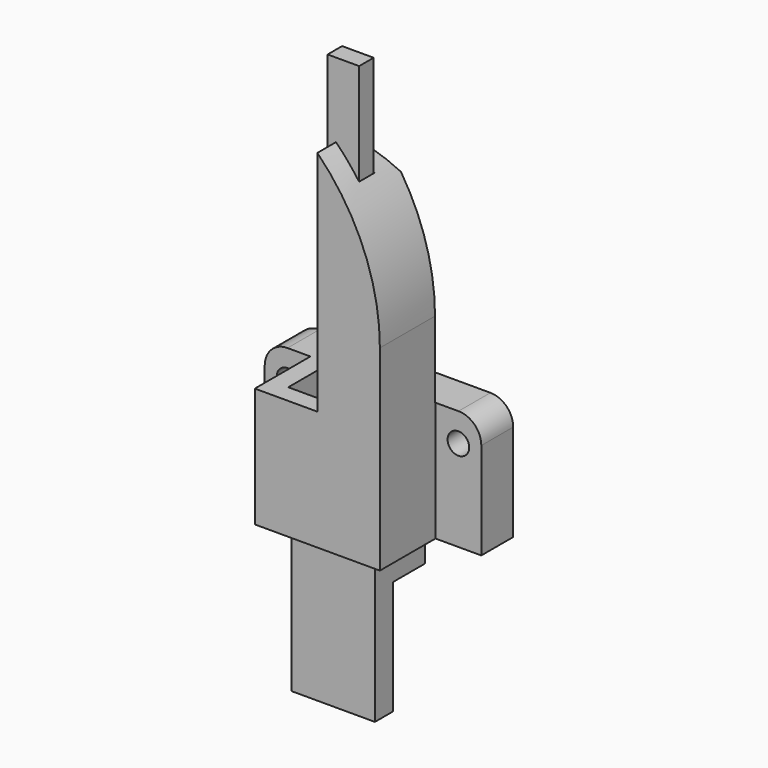
from build123d import *

# Parameters (mm, degrees)
F0_W         = 18.542
F0_H         = 8.89
F1_DEPTH     = 6.35
F2_DEPTH     = 5.08
F3_W         = 18.542
F3_H         = 5.0685656011
F4_DEPTH     = 25.4
F5_W         = 7.493
F5_H         = 4.191
F6_DEPTH     = 125.222
F7_DEPTH     = 6.35
F8_W         = 7.0358
F8_H         = 4.0401988663
F9_DEPTH     = 127
F11_DEPTH    = 21.59
F12_R        = 2.413
F13_DEPTH    = 25.4
F14_W        = 19.3073768169
F14_H        = 14.7933904082
F15_DEPTH    = 41.656
F16_W        = 10.1808982092
F16_H        = 21.59
F16_W_2      = 10.2163404226
F17_DEPTH    = 15.494
F18_DEPTH    = 5.08
F19_DEPTH    = 6.35
F20_W        = 13.9391366392
F20_H        = 15.3644406528
F21_DEPTH    = 50.8
F22_T1_DEPTH = 184.1193966406
F23_SIZE     = 6.35
F24_R        = 5.08
F25_W        = 7.1110432036
F25_H        = 4.2591807432
F26_DEPTH    = 73.152
F27_DEPTH    = 4.445
F28_R        = 2.54
F30_DEPTH    = 25.4
F29_R        = 3.937
F31_DEPTH    = 11.43


# Not quite as in the source:
# - a fillet or chamfer that OpenCascade refuses, or shapes differently, is made with other operations: its cross-section is extruded or revolved along the edge and cut away or added


with BuildPart() as f1:
    # F0 (on Top) → F1 (new body)
    with BuildSketch(Plane.XY):
        Rectangle(F0_W, F0_H)
    extrude(amount=F1_DEPTH)

    # F2 (add): a face of the model
    f2_faces = [f1.faces().sort_by_distance(p)[0] for p in [
        (0, -4.445, 3.175),
    ]]
    extrude(f2_faces, amount=F2_DEPTH)

    # F3 (on face) → F4 (join)
    with BuildSketch(Plane(origin=(0, 0, 0), x_dir=(1, 0, 0), z_dir=(0, 0, -1))):
        with Locations((0, 6.9907171994)):
            Rectangle(F3_W, F3_H)
    extrude(amount=F4_DEPTH)

    # F5 (on face) → F6 (cut)
    with BuildSketch(Plane(origin=(0, 0, -25.4), x_dir=(1, 0, 0), z_dir=(0, 0, -1))):
        with Locations((1.6165795822, 6.5519343989)):
            Rectangle(F5_W, F5_H)
    extrude(amount=-F6_DEPTH, mode=Mode.SUBTRACT)

    # F7 (add): a face of the model
    f7_faces = [f1.faces().sort_by_distance(p)[0] for p in [
        (-0.2230199424, -1.9865219107, 6.35),
    ]]
    extrude(f7_faces, amount=F7_DEPTH)

    # F19 (add): a face of the model
    f19_faces = [f1.faces().sort_by_distance(p)[0] for p in [
        (-0.2230199424, -1.9865219107, 12.7),
    ]]
    extrude(f19_faces, amount=F19_DEPTH)

    # F28 (on face) → F30 (cut)
    with BuildSketch(Plane.XY.offset(19.05)):
        Circle(F28_R)
    extrude(amount=-F30_DEPTH, mode=Mode.SUBTRACT)

    # F29 (on face) → F31 (cut)
    with BuildSketch(Plane.XY.offset(19.05)):
        Circle(F29_R)
    extrude(amount=-F31_DEPTH, mode=Mode.SUBTRACT)


with BuildPart() as f9:
    # F8 (on face) → F9 (new body)
    with BuildSketch(Plane(origin=(0, 0, -25.4), x_dir=(1, 0, 0), z_dir=(0, 0, -1))):
        with Locations((1.5412379404, 6.6265871283)):
            Rectangle(F8_W, F8_H)
    extrude(amount=-F9_DEPTH)


with BuildPart() as f11:
    # F10 (on face) → F11 (new body)
    with BuildSketch(Plane.XY.offset(12.7)):
        Polygon((-24.13, 5.969), (-24.13, 0), (-24.13, -13.97), (24.1554770619, -13.97), (24.1554770619, 5.969), align=None)
    extrude(amount=F11_DEPTH)

    # F12 (on face) → F13 (cut)
    with BuildSketch(Plane(origin=(0, 5.969, 0), x_dir=(-1, 0, 0), z_dir=(0, 1, 0))):
        with Locations((19.05, 27.94)):
            Circle(F12_R)
        with Locations((-19.05, 27.94)):
            Circle(F12_R)
    extrude(amount=-F13_DEPTH, mode=Mode.SUBTRACT)

    # F14 (on face) → F15 (cut)
    with BuildSketch(Plane(origin=(0, 0, 12.7), x_dir=(1, 0, 0), z_dir=(0, 0, -1))):
        with Locations((-0.0584181398, 2.5467472151)):
            Rectangle(F14_W, F14_H)
    extrude(amount=-F15_DEPTH, mode=Mode.SUBTRACT)

    # F16 (on face) → F17 (cut)
    with BuildSketch(Plane.XZ.offset(13.97)):
        with Locations((-19.0395508954, 23.495)):
            Rectangle(F16_W, F16_H)
        with Locations((19.0473068506, 23.495)):
            Rectangle(F16_W_2, F16_H)
    extrude(amount=-F17_DEPTH, mode=Mode.SUBTRACT)

    # F18 (add): a face of the model
    f18_faces = [f11.faces().sort_by_distance(p)[0] for p in [
        (19.0473068506, 2.0464031983, 12.7),
    ]]
    extrude(f18_faces, amount=F18_DEPTH)

    # F20 (on face) → F21 (join)
    with BuildSketch(Plane.XY.offset(34.29)):
        with Locations((6.9695683196, -6.2877796736)):
            Rectangle(F20_W, F20_H)
    extrude(amount=F21_DEPTH)

    # F22: fillet of radius 47.8303990977 on 1 edges, made by hand

    # F22_s2 → F22_t1 (cut)
    with BuildSketch(Plane.XZ.offset(-85.7719186467)):
        with BuildLine():
            ThreePointArc((0, 85.09), (10.3172191212, 69.5970819282), (13.9391366392, 51.3390088024))
            Line((13.9391366392, 51.3390088024), (13.9391366392, 85.09))
            Line((13.9391366392, 85.09), (0, 85.09))
        make_face()
    extrude(amount=F22_T1_DEPTH, mode=Mode.SUBTRACT)

    # F23
    f23_edges = [f11.edges().sort_by_distance(p)[0] for p in [
        (0, 1.394441, 59.69),
    ]]
    chamfer(f23_edges, length=F23_SIZE)

    # F24
    f24_edges = [f11.edges().sort_by_distance(p)[0] for p in [
        (-24.13, 3.7465, 34.29),
        (24.155477, 3.7465, 34.29),
    ]]
    fillet(f24_edges, radius=F24_R)

    # F25 (on face) → F26 (cut)
    with BuildSketch(Plane.XY.offset(34.29)):
        with Locations((1.5899057034, -6.6439488437)):
            Rectangle(F25_W, F25_H)
    extrude(amount=F26_DEPTH, mode=Mode.SUBTRACT)

    # F27 (add): a face of the model
    f27_faces = [f11.faces().sort_by_distance(p)[0] for p in [
        (0.0131143273, 5.969, 20.6399690169),
    ]]
    extrude(f27_faces, amount=F27_DEPTH)


solid = Compound([f1.part, f9.part, f11.part])
